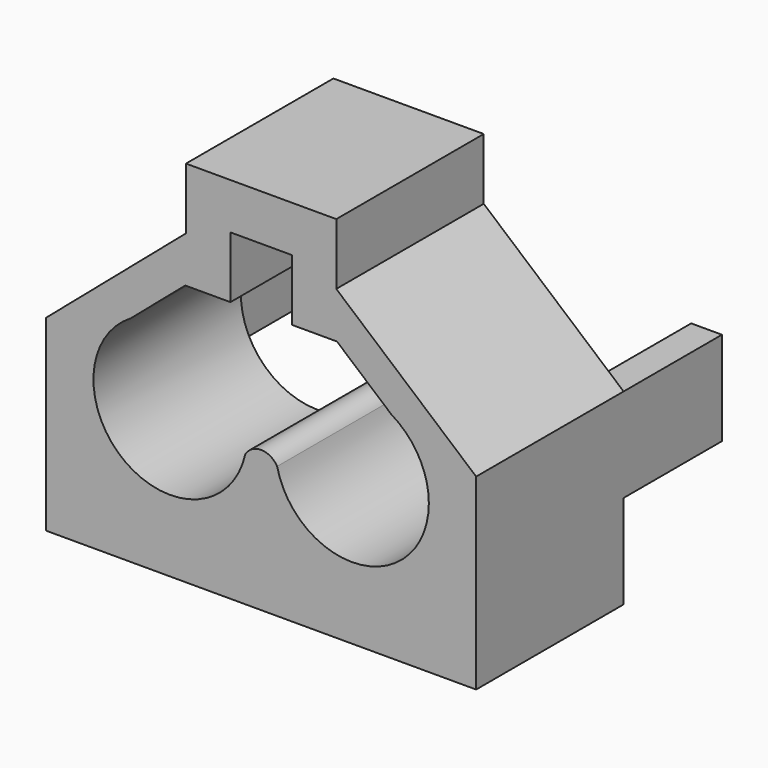
from build123d import *

# Parameters (mm, degrees)
F1_DEPTH = 19.05
F2_W     = 3.175
F2_H     = 9.6882774726
F3_DEPTH = 12.7


# Not quite as in the source:
# - ends of sketch curves that miss each other by under 0.0002 mm in the source are joined


with BuildPart() as f1:
    # F0 (on Front) → F1 (new body)
    with BuildSketch(Plane.XZ):
        Polygon((-7.493, 0.1328983575), (0, 0.1328983575), (7.493, 0.1328983575), (22.2194990303, 0.1328983575), (22.2194990303, 19.5094533027), (7.7658264293, 31.8828983575), (7.7658264293, 38.2328983575), (-7.7713273633, 38.2328983575), (-7.7713273633, 31.8828983575), (-22.2249999642, 19.5094533027), (-22.2249999642, 4.5234533027), (-22.2249999642, 0.1328983575), align=None)
        with BuildLine():
            ThreePointArc((-1.6471995105, 13.7654938087), (-14.0416307026, 9.056743723), (-13.4701421127, 22.3031640975))
            Line((-13.4701421127, 22.3031640975), (-7.8430329322, 27.1203983575))
            Line((-7.8430329322, 27.1203983575), (-3.175, 27.1203983575))
            Line((-3.175, 27.1203983575), (-3.175, 30.2953983575))
            Line((-3.175, 30.2953983575), (-3.175, 33.4703983575))
            Line((-3.175, 33.4703983575), (3.175, 33.4703983575))
            Line((3.175, 33.4703983575), (3.175, 30.2953983575))
            Line((3.175, 30.2953983575), (3.175, 27.1203983575))
            Line((3.175, 27.1203983575), (7.8375319983, 27.1203983575))
            Line((7.8375319983, 27.1203983575), (13.4701421127, 22.3031640975))
            ThreePointArc((13.4701421127, 22.3031640975), (16.2995077669, 19.40684068), (17.3322006389, 15.4917998403))
            ThreePointArc((17.3322006389, 15.4917998403), (10.2711150187, 7.6028326022), (1.6507381924, 13.7496885133))
            ThreePointArc((1.6507381924, 13.7496885133), (0.0063534061, 14.7141035739), (-1.6471995105, 13.7654938087))
        make_face(mode=Mode.SUBTRACT)
    extrude(amount=F1_DEPTH)

    # F2 (on face) → F3 (join)
    with BuildSketch(Plane(origin=(0, 0, 0), x_dir=(-1, 0, 0), z_dir=(0, 1, 0))):
        with Locations((-20.6319990303, 14.6653145664)):
            Rectangle(F2_W, F2_H)
        with Locations((20.6374999642, 14.6653145664)):
            Rectangle(F2_W, F2_H)
        Polygon((-4.239049533, 3.3078983575), (-4.239049533, 0.1328983575), (0.002750467, 0.1328983575), (4.244550467, 0.1328983575), (4.244550467, 3.3078983575), align=None)
    extrude(amount=F3_DEPTH)


solid = f1.part
